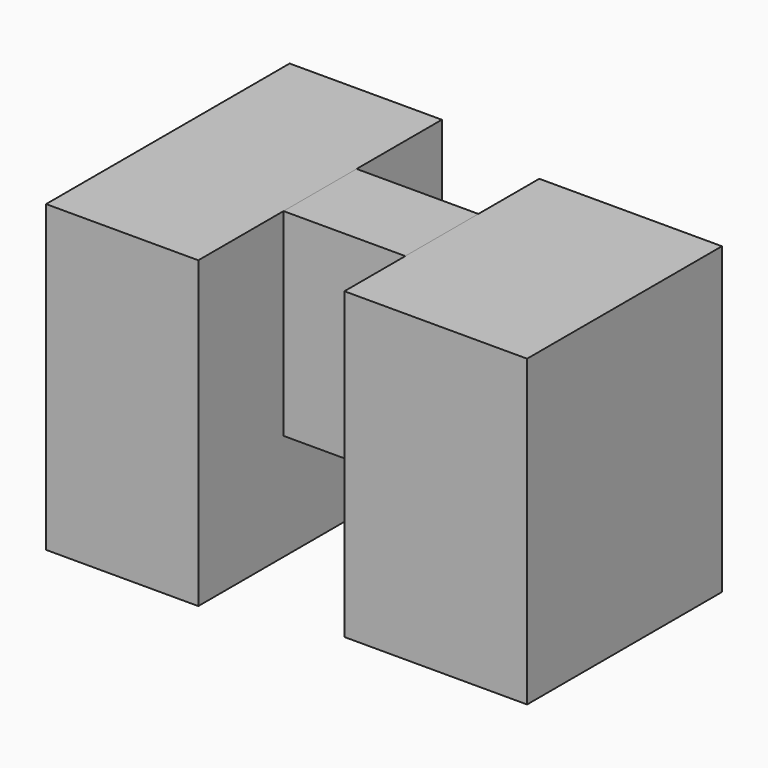
from build123d import *

# Parameters (mm, degrees)
F0_W     = 50
F0_H     = 100
F1_DEPTH = 100
F2_W     = 30
F2_H     = 65
F3_DEPTH = 40
F4_W     = 80
F4_H     = 100
F5_DEPTH = 60
F6_W     = 17.1575322747
F6_H     = 26.2599568814
F7_DEPTH = 25
F9_DEPTH = 17.1575322747


with BuildPart() as f1:
    # F0 (on Top) → F1 (new body)
    with BuildSketch(Plane.XY):
        with Locations((25, 50)):
            Rectangle(F0_W, F0_H)
    extrude(amount=F1_DEPTH)


with BuildPart() as f3:
    # F2 (on face) → F3 (new body)
    with BuildSketch(Plane.YZ.offset(50)):
        with Locations((50, 67.5)):
            Rectangle(F2_W, F2_H)
    extrude(amount=F3_DEPTH)


with BuildPart() as f5:
    # F4 (on face) → F5 (new body)
    with BuildSketch(Plane.YZ.offset(90)):
        with Locations((50, 50)):
            Rectangle(F4_W, F4_H)
    extrude(amount=F5_DEPTH)


with BuildPart() as f7:
    # F6 (on Top) → F7 (new body)
    with BuildSketch(Plane.XY):
        with Locations((122.7362714708, 39.2065504566)):
            Rectangle(F6_W, F6_H)
    extrude(amount=F7_DEPTH)

    # F8 (on face) → F9 (cut, through all)
    with BuildSketch(Plane.YZ.offset(131.3150376081)):
        Polygon((52.3365288973, 25), (39.2065504566, 25), (39.2065504566, 10.100197047), (46.3397689164, 10.100197047), (46.3397689164, 5.4961908609), (52.3365288973, 5.4961908609), align=None)
    extrude(amount=-F9_DEPTH, mode=Mode.SUBTRACT)


solid = Compound([f1.part, f3.part, f5.part, f7.part])
